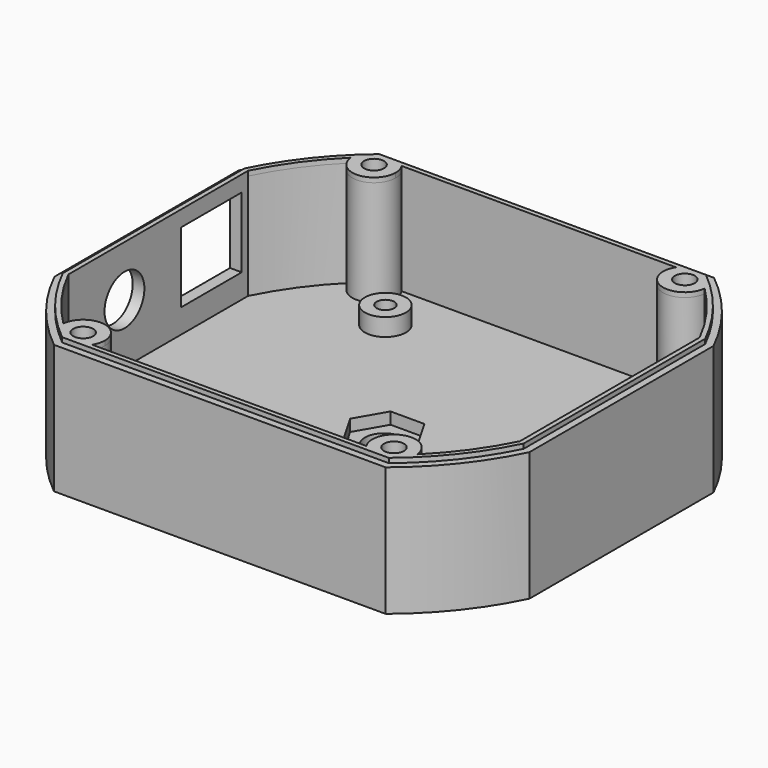
from build123d import *

# Parameters (mm, degrees)
F0_R      = 1.7
F1_DEPTH  = 22
F2_T      = -2
F3_SIZE   = 1.4
F4_R      = 1.7
F5_DEPTH  = 0.8
F6_R      = 3.5
F6_R_2    = 1.5
F7_DEPTH  = 5
F8_W      = 13
F8_H      = 12
F8_R      = 4.25
F9_DEPTH  = 2
F10_R     = 3.5
F11_DEPTH = 2
F12_D     = 6.5


# Not quite as in the source:
# - a feature names something its author has since deleted; it is built from what else it names


with BuildPart() as f1:
    # F0 (on Top) → F1 (new body)
    with BuildSketch(Plane.XY):
        with BuildLine():
            Line((-40.5, 19.6150452459), (-40.5, -19.6150452459))
            ThreePointArc((-40.5, -19.6150452459), (-35.2419239111, -27.982258648), (-28.2842712475, -35))
            Line((-28.2842712475, -35), (28.2842712475, -35))
            ThreePointArc((28.2842712475, -35), (35.2419239111, -27.982258648), (40.5, -19.6150452459))
            Line((40.5, -19.6150452459), (40.5, 19.6150452459))
            ThreePointArc((40.5, 19.6150452459), (35.2419239111, 27.982258648), (28.2842712475, 35))
            Line((28.2842712475, 35), (-28.2842712475, 35))
            ThreePointArc((-28.2842712475, 35), (-35.2419239111, 27.982258648), (-40.5, 19.6150452459))
        make_face()
        with Locations((-26.5, -31)):
            Circle(F0_R, mode=Mode.SUBTRACT)
        with Locations((26.5, -31)):
            Circle(F0_R, mode=Mode.SUBTRACT)
        with Locations((-26.5, 31)):
            Circle(F0_R, mode=Mode.SUBTRACT)
        with Locations((26.5, 31)):
            Circle(F0_R, mode=Mode.SUBTRACT)
    extrude(amount=F1_DEPTH)

    # F2
    f2_openings = [f1.faces().sort_by_distance(p)[0] for p in [
        (0, 0, 22),
    ]]
    offset(amount=F2_T, openings=f2_openings)

    # F3
    f3_edges = [f1.edges().sort_by_distance(p)[0] for p in [
        (-28.2, -31, 0),
        (24.8, -31, 0),
        (24.8, 31, 0),
        (-28.2, 31, 0),
    ]]
    chamfer(f3_edges, length=F3_SIZE)

    # F4 (on face) → F5 (join)
    with BuildSketch(Plane.XY.offset(22)):
        with BuildLine():
            Line((27.8567765544, 33.8), (-27.8567765544, 33.8))
            ThreePointArc((-27.8567765544, 33.8), (-34.3481740656, 27.1779862823), (-39.3, 19.3377868434))
            Line((-39.3, 19.3377868434), (-39.3, -19.3377868434))
            ThreePointArc((-39.3, -19.3377868434), (-34.3481740656, -27.1779862823), (-27.8567765544, -33.8))
            Line((-27.8567765544, -33.8), (27.8567765544, -33.8))
            ThreePointArc((27.8567765544, -33.8), (34.3481740656, -27.1779862823), (39.3, -19.3377868434))
            Line((39.3, -19.3377868434), (39.3, 19.3377868434))
            ThreePointArc((39.3, 19.3377868434), (34.3481740656, 27.1779862823), (27.8567765544, 33.8))
        make_face()
        with Locations((-26.5, -31)):
            Circle(F4_R, mode=Mode.SUBTRACT)
        with Locations((26.5, -31)):
            Circle(F4_R, mode=Mode.SUBTRACT)
        with Locations((-26.5, 31)):
            Circle(F4_R, mode=Mode.SUBTRACT)
        with BuildLine():
            ThreePointArc((30.1812784263, -30.6282619904), (25.2805511537, -27.5067286806), (23.3871235167, -33))
            Line((23.3871235167, -33), (-23.3871235167, -33))
            ThreePointArc((-23.3871235167, -33), (-22.949813879, -32.0421988802), (-22.8, -31))
            ThreePointArc((-22.8, -31), (-26.3138954292, -27.3046833574), (-30.1812784263, -30.6282619904))
            ThreePointArc((-30.1812784263, -30.6282619904), (-34.8168494492, -25.2346387815), (-38.5, -19.1507180022))
            Line((-38.5, -19.1507180022), (-38.5, 19.1507180022))
            ThreePointArc((-38.5, 19.1507180022), (-34.8168494492, 25.2346387815), (-30.1812784263, 30.6282619904))
            ThreePointArc((-30.1812784263, 30.6282619904), (-26.3138954292, 27.3046833574), (-22.8, 31))
            ThreePointArc((-22.8, 31), (-22.949813879, 32.0421988802), (-23.3871235167, 33))
            Line((-23.3871235167, 33), (23.3871235167, 33))
            ThreePointArc((23.3871235167, 33), (25.2805511537, 27.5067286806), (30.1812784263, 30.6282619904))
            ThreePointArc((30.1812784263, 30.6282619904), (34.8168494492, 25.2346387815), (38.5, 19.1507180022))
            Line((38.5, 19.1507180022), (38.5, -19.1507180022))
            ThreePointArc((38.5, -19.1507180022), (34.8168494492, -25.2346387815), (30.1812784263, -30.6282619904))
        make_face(mode=Mode.SUBTRACT)
        with Locations((26.5, 31)):
            Circle(F4_R, mode=Mode.SUBTRACT)
    extrude(amount=F5_DEPTH)

    # F6 (on face) → F7 (join)
    with BuildSketch(Plane.XY.offset(2)):
        with Locations((-19, 24.05)):
            Circle(F6_R)
        with Locations((-19, 24.05)):
            Circle(F6_R_2, mode=Mode.SUBTRACT)
        with Locations((31.8, 8.85)):
            Circle(F6_R)
        with Locations((31.8, 8.85)):
            Circle(F6_R_2, mode=Mode.SUBTRACT)
        with Locations((31.8, -19.05)):
            Circle(F6_R)
        with Locations((31.8, -19.05)):
            Circle(F6_R_2, mode=Mode.SUBTRACT)
        with Locations((-20.3, -24.15)):
            Circle(F6_R)
        with Locations((-20.3, -24.15)):
            Circle(F6_R_2, mode=Mode.SUBTRACT)
    extrude(amount=F7_DEPTH)

    # F8 (on face) → F9 (cut, through all)
    with BuildSketch(Plane(origin=(-40.5, 0, 0), x_dir=(0, -1, 0), z_dir=(-1, 0, 0))):
        with Locations((-11.3, 14.1)):
            Rectangle(F8_W, F8_H)
        with Locations((7.2, 14.1)):
            Circle(F8_R)
    extrude(amount=-F9_DEPTH, mode=Mode.SUBTRACT)

    # F10 (on face) → F11 (join)
    with BuildSketch(Plane.XY.offset(2)):
        with BuildLine():
            ThreePointArc((-23.3871235167, 33), (-25.2805511537, 27.5067286806), (-30.1812784263, 30.6282619904))
            ThreePointArc((-30.1812784263, 30.6282619904), (-34.8168494492, 25.2346387815), (-38.5, 19.1507180022))
            Line((-38.5, 19.1507180022), (-38.5, -19.1507180022))
            ThreePointArc((-38.5, -19.1507180022), (-34.8168494492, -25.2346387815), (-30.1812784263, -30.6282619904))
            ThreePointArc((-30.1812784263, -30.6282619904), (-25.2805511537, -27.5067286806), (-23.3871235167, -33))
            Line((-23.3871235167, -33), (23.3871235167, -33))
            ThreePointArc((23.3871235167, -33), (25.2805511537, -27.5067286806), (30.1812784263, -30.6282619904))
            ThreePointArc((30.1812784263, -30.6282619904), (34.8168494492, -25.2346387815), (38.5, -19.1507180022))
            Line((38.5, -19.1507180022), (38.5, 19.1507180022))
            ThreePointArc((38.5, 19.1507180022), (34.8168494492, 25.2346387815), (30.1812784263, 30.6282619904))
            ThreePointArc((30.1812784263, 30.6282619904), (25.2805511537, 27.5067286806), (23.3871235167, 33))
            Line((23.3871235167, 33), (-23.3871235167, 33))
        make_face()
        with Locations((-20.3, -24.15)):
            Circle(F10_R, mode=Mode.SUBTRACT)
        with Locations((31.8, -19.05)):
            Circle(F10_R, mode=Mode.SUBTRACT)
        with Locations((-19, 24.05)):
            Circle(F10_R, mode=Mode.SUBTRACT)
        Polygon((-5.7735026919, 0), (-2.8867513459, 5), (2.8867513459, 5), (5.7735026919, 0), (2.8867513459, -5), (-2.8867513459, -5), align=None, mode=Mode.SUBTRACT)
        with Locations((31.8, 8.85)):
            Circle(F10_R, mode=Mode.SUBTRACT)
    extrude(amount=F11_DEPTH)

    # F12 (through all)
    with Locations(Plane.XY.offset(2)):
        with Locations((0, 0)):
            Hole(F12_D / 2)


solid = f1.part
